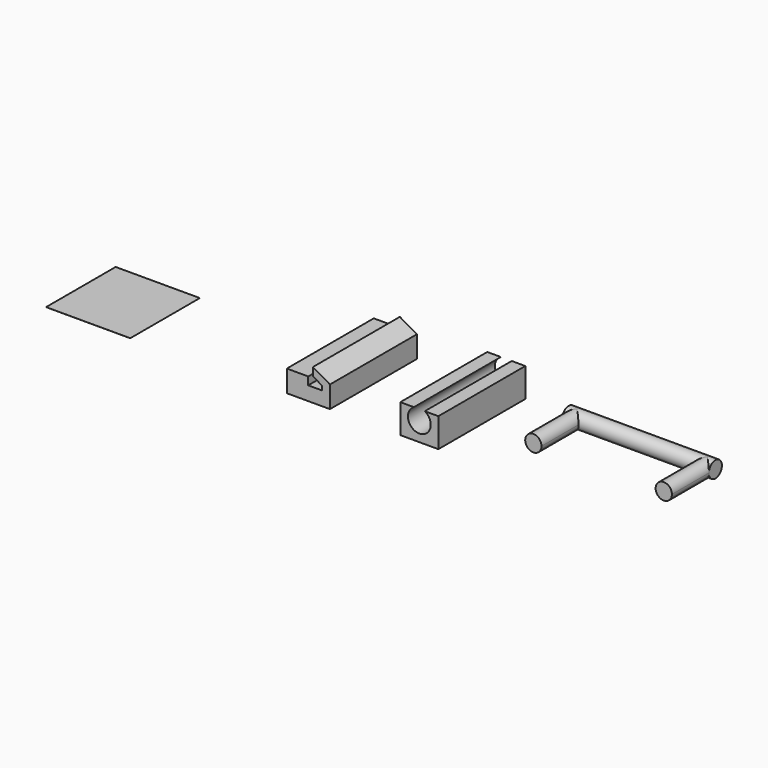
from build123d import *
from build123d import SkipClean  # not in build123d's __all__

# Parameters (mm, degrees)
F1_DEPTH    = 10
F2_W        = 7.7500019912
F2_H        = 8
F3_DEPTH    = 1
F4_T1_DEPTH = 22.7500019912
F4_T3_DEPTH = 23
F6_DEPTH    = 10
F8_DEPTH    = 5


# Not quite as in the source:
# - a fillet or chamfer that OpenCascade refuses, or shapes differently, is made with other operations: its cross-section is extruded or revolved along the edge and cut away or added


with BuildPart() as f1:
    # F0 (on Front) → F1 (new body)
    with BuildSketch(Plane.XZ):
        Polygon((3.4554570526, 2), (1.4884697545, 2), (1.4884697545, 0), (5.4554570526, 0), (5.4554570526, 2), (3.8884697545, 2.9047005384), (3.8884697545, 2.1547005384), (4.1564189469, 2), (4.7054570526, 1.6830127019), (4.7054570526, 1.2783121635), (3.8884697545, 1.2783121635), (3.4554570526, 1.2783121635), align=None)
    extrude(amount=F1_DEPTH)


with BuildPart() as f3:
    # F2 (on Top) → F3 (new body)
    with BuildSketch(Plane.XY):
        with Locations((-15.3153333813, -7.8402892686)):
            Rectangle(F2_W, F2_H)
    extrude(amount=F3_DEPTH)

    # F4: fillet of radius 5 on 4 edges, made by hand

    # F4_s2 → F4_t1 (cut)
    with BuildSketch(Plane.YZ.offset(-26.6903343769)):
        with BuildLine():
            ThreePointArc((-3.8402892686, 1), (-5.2591504386, 0.2565835097), (-6.8402892686, 0))
            Line((-6.8402892686, 0), (-6.8402892686, -0.1))
            Line((-6.8402892686, -0.1), (-3.8402892686, -0.1))
            Line((-3.8402892686, -0.1), (-3.7402892686, 0))
            ThreePointArc((-3.7402892686, 0), (-3.7402892686, 0.5), (-3.7802892686, 0.92))
            Line((-3.7802892686, 0.92), (-3.8402892686, 1))
        make_face()
        with BuildLine():
            ThreePointArc((-11.8402892686, 1), (-10.4214280987, 0.2565835097), (-8.8402892686, 0))
            Line((-8.8402892686, 0), (-8.8402892686, -0.1))
            Line((-8.8402892686, -0.1), (-11.8402892686, -0.1))
            Line((-11.8402892686, -0.1), (-11.9402892686, 0))
            ThreePointArc((-11.9402892686, 0), (-11.9402892686, 0.5), (-11.9002892686, 0.92))
            Line((-11.9002892686, 0.92), (-11.8402892686, 1))
        make_face()
    extrude(amount=F4_T1_DEPTH, mode=Mode.SUBTRACT)

    # F4_s4 → F4_t3 (cut)
    with BuildSketch(Plane.XZ.offset(-3.6597107314)):
        with BuildLine():
            ThreePointArc((-19.1903343769, 1), (-17.771473207, 0.2565835097), (-16.1903343769, 0))
            Line((-16.1903343769, 0), (-16.1903343769, -0.1))
            Line((-16.1903343769, -0.1), (-19.1903343769, -0.1))
            Line((-19.1903343769, -0.1), (-19.2903343769, 0))
            ThreePointArc((-19.2903343769, 0), (-19.2903343769, 0.5), (-19.2503343769, 0.92))
            Line((-19.2503343769, 0.92), (-19.1903343769, 1))
        make_face()
        with BuildLine():
            ThreePointArc((-11.4403323857, 1), (-12.8591935556, 0.2565835097), (-14.4403323857, 0))
            Line((-14.4403323857, 0), (-14.4403323857, -0.1))
            Line((-14.4403323857, -0.1), (-11.4403323857, -0.1))
            Line((-11.4403323857, -0.1), (-11.3403323857, 0))
            ThreePointArc((-11.3403323857, 0), (-11.3403323857, 0.5), (-11.3803323857, 0.92))
            Line((-11.3803323857, 0.92), (-11.4403323857, 1))
        make_face()
    extrude(amount=F4_T3_DEPTH, mode=Mode.SUBTRACT)


with BuildPart() as f6:
    # F5 (on Front) → F6 (new body)
    with BuildSketch(Plane.XZ):
        with BuildLine():
            Line((13.1807962247, 2.6733092656), (11.9307962247, 2.6733092656))
            Line((11.9307962247, 2.6733092656), (11.9307962247, 0))
            Line((11.9307962247, 0), (15.4307962247, 0))
            Line((15.4307962247, 0), (15.4307962247, 2.6733092656))
            Line((15.4307962247, 2.6733092656), (14.1807962247, 2.6733092656))
            ThreePointArc((14.1807962247, 2.6733092656), (14.5828771524, 2.2873546315), (14.7307962247, 1.75))
            ThreePointArc((14.7307962247, 1.75), (13.1434415932, 0.8479190724), (13.1807962247, 2.6733092656))
        make_face()
    extrude(amount=F6_DEPTH)


with BuildPart() as f8:
    # F7 (on Front) → F8 (new body)
    with BuildSketch(Plane.XZ):
        with BuildLine():
            ThreePointArc((20.1727531818, -0.75), (20.7030832677, -0.5303300859), (20.9227531818, 0))
            Line((20.9227531818, 0), (19.4227531818, 0))
            ThreePointArc((19.4227531818, 0), (19.6424230959, -0.5303300859), (20.1727531818, -0.75))
        make_face()
        with BuildLine():
            Line((19.4227531818, 0), (20.9227531818, 0))
            ThreePointArc((20.9227531818, 0), (20.1727531818, 0.75), (19.4227531818, 0))
        make_face()
    extrude(amount=F8_DEPTH)



with BuildPart() as f8b:
    # F7 (on Front) → F8, piece 2 (new body)
    with BuildSketch(Plane.XZ):
        with BuildLine():
            ThreePointArc((32.1727531818, -0.75), (32.7030832677, -0.5303300859), (32.9227531818, 0))
            Line((32.9227531818, 0), (31.4227531818, 0))
            ThreePointArc((31.4227531818, 0), (31.6424230959, -0.5303300859), (32.1727531818, -0.75))
        make_face()
        with BuildLine():
            Line((31.4227531818, 0), (32.9227531818, 0))
            ThreePointArc((32.9227531818, 0), (32.1727531818, 0.75), (31.4227531818, 0))
        make_face()
    extrude(amount=F8_DEPTH)


with BuildPart() as f8_1:
    add(f8.part, clean=False)

    with SkipClean():  # cleaning this boolean's faces spoils the solid; the shape is the same uncleaned
        add(f8b.part)  # F9 merges F8b
    # F7 (on Front) → F9 (revolve)
    with BuildSketch(Plane.XZ):
        with BuildLine():
            Line((32.9227531818, -0.75), (32.9227531818, 0))
            ThreePointArc((32.9227531818, 0), (32.7030832677, -0.5303300859), (32.1727531818, -0.75))
            Line((32.1727531818, -0.75), (32.9227531818, -0.75))
        make_face()
        with BuildLine():
            ThreePointArc((32.1727531818, -0.75), (32.7030832677, -0.5303300859), (32.9227531818, 0))
            Line((32.9227531818, 0), (31.4227531818, 0))
            ThreePointArc((31.4227531818, 0), (31.6424230959, -0.5303300859), (32.1727531818, -0.75))
        make_face()
        with BuildLine():
            ThreePointArc((32.1727531818, -0.75), (31.6424230959, -0.5303300859), (31.4227531818, 0))
            Line((31.4227531818, 0), (20.9227531818, 0))
            ThreePointArc((20.9227531818, 0), (20.7030832677, -0.5303300859), (20.1727531818, -0.75))
            Line((20.1727531818, -0.75), (32.1727531818, -0.75))
        make_face()
        with BuildLine():
            ThreePointArc((20.1727531818, -0.75), (20.7030832677, -0.5303300859), (20.9227531818, 0))
            Line((20.9227531818, 0), (19.4227531818, 0))
            ThreePointArc((19.4227531818, 0), (19.6424230959, -0.5303300859), (20.1727531818, -0.75))
        make_face()
        with BuildLine():
            Line((19.4227531818, -0.75), (20.1727531818, -0.75))
            ThreePointArc((20.1727531818, -0.75), (19.6424230959, -0.5303300859), (19.4227531818, 0))
            Line((19.4227531818, 0), (19.4227531818, -0.75))
        make_face()
    with SkipClean():  # cleaning this boolean's faces spoils the solid; the shape is the same uncleaned
        revolve(axis=Axis((26.1727531818, 0, 0), (-1, 0, 0)))


solid = Compound([f1.part, f3.part, f6.part, f8_1.part])
